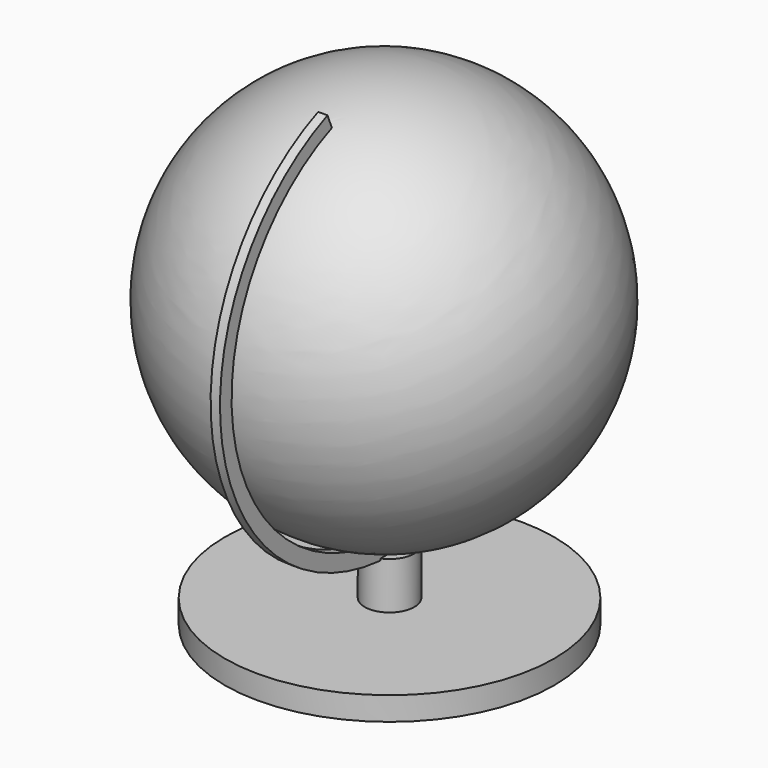
from build123d import *

# Parameters (mm, degrees)
F0_R     = 44.471703747
F1_DEPTH = 6.35
F2_R     = 6.7051152742
F3_DEPTH = 12.7
F5_DEPTH = 2.54


with BuildPart() as f1:
    # F0 (on Top) → F1 (new body)
    with BuildSketch(Plane.XY):
        Circle(F0_R)
    extrude(amount=F1_DEPTH)

    # F2 (on face) → F3 (join)
    with BuildSketch(Plane.XY.offset(6.35)):
        Circle(F2_R)
    extrude(amount=F3_DEPTH)

    # F4 (on Right) → F5 (join)
    with BuildSketch(Plane.YZ):
        with BuildLine():
            Line((-22.6401387629, 128.1149116989), (-24.116454646, 131.6991597414))
            ThreePointArc((-24.116454646, 131.6991597414), (-55.9675009555, 54.8518749978), (20.7669115572, 22.7298535827))
            Line((20.7669115572, 22.7298535827), (19.0143249929, 26.9848406315))
            ThreePointArc((19.0143249929, 26.9848406315), (-52.3779424187, 56.7226442873), (-22.6401387629, 128.1149116989))
        make_face()
    extrude(amount=F5_DEPTH)


with BuildPart() as f7:
    # F6 (on Right) → F7 (revolve)
    with BuildSketch(Plane.YZ):
        with BuildLine():
            Line((18.5737852007, 27.7495793998), (-22.3302803934, 127.9227882624))
            ThreePointArc((-22.3302803934, 127.9227882624), (-51.3615475217, 57.6305004059), (18.5737852007, 27.7495793998))
        make_face()
    revolve(axis=Axis((0, -1.8782475963, 77.8361838311), (0, 0.3780319987, -0.9257925297)))


solid = Compound([f1.part, f7.part])
